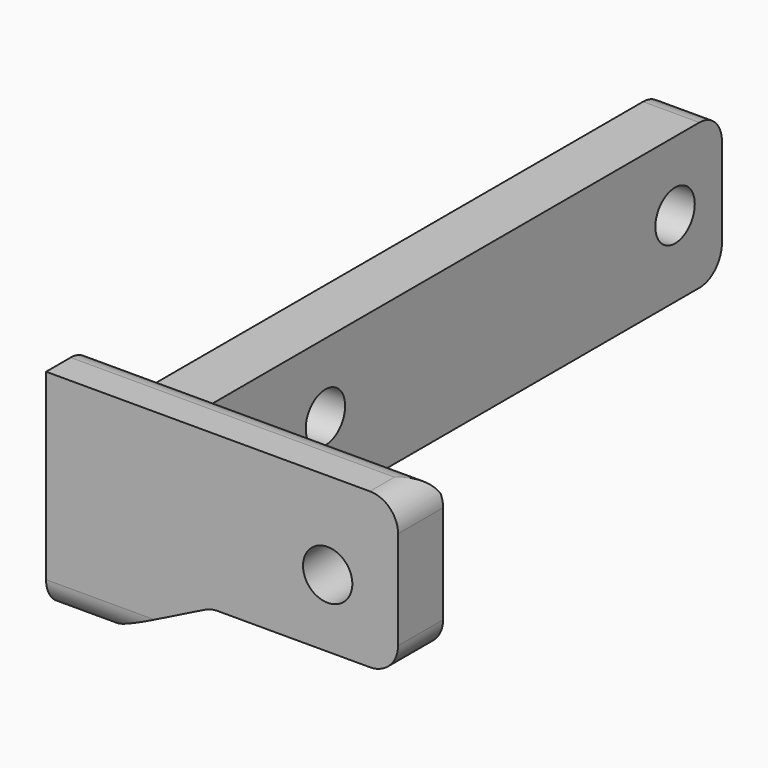
from build123d import *

# Parameters (mm, degrees)
F0_W         = 4
F0_H         = 51
F0_H_2       = 4
F0_W_2       = 21
F1_DEPTH     = 15
F4_D         = 3.5
F4_ON_F3_D   = 3.5
F5_DEPTH     = 25
F6_DEPTH     = 25
F7_T1_DEPTH  = 4
F7_T3_DEPTH  = 14
F7_T5_DEPTH  = 13.3694414049
F7_T7_DEPTH  = 14
F7_T9_DEPTH  = 30.9469097591
F7_T11_DEPTH = 13.6920837807


# Not quite as in the source:
# - a fillet or chamfer that OpenCascade refuses, or shapes differently, is made with other operations: its cross-section is extruded or revolved along the edge and cut away or added


with BuildPart() as f1:
    # F0 (on Top) → F1 (new body)
    with BuildSketch(Plane.XY):
        with Locations((0, 2)):
            Rectangle(F0_W, F0_H)
        with Locations((0, -25.5)):
            Rectangle(F0_W, F0_H_2)
        with Locations((12.5, -25.5)):
            Rectangle(F0_W_2, F0_H_2)
    extrude(amount=F1_DEPTH)

    # F4 (through all)
    with Locations(Plane(origin=(-2, 0, 0), x_dir=(0, -1, 0), z_dir=(-1, 0, 0))):
        with Locations((-23.34, 5.4024579003), (7.7, 5.4024579003)):
            Hole(F4_D / 2)

    # F4 on F3 (through all)
    with Locations(Plane.XZ.offset(27.5)):
        with Locations((18, 8.8024579003)):
            Hole(F4_ON_F3_D / 2)

    # F2 (on face) → F5 (cut)
    with BuildSketch(Plane(origin=(-2, 0, 0), x_dir=(0, -1, 0), z_dir=(-1, 0, 0))):
        Polygon((-27.5, 15), (-27.5, 10.3389231786), (21.5976021229, 10.3389231786), (24.1305585951, 15), align=None)
    extrude(amount=-F5_DEPTH, mode=Mode.SUBTRACT)

    # F3 (on face) → F6 (cut)
    with BuildSketch(Plane.XZ.offset(27.5)):
        Polygon((23, 0), (23, 4), (9.7110802308, 4), (1.6920837807, 0), align=None)
    extrude(amount=-F6_DEPTH, mode=Mode.SUBTRACT)

    # F7: fillet of radius 2 on 7 edges, made by hand

    # F7_s2 → F7_t1 (join)
    with BuildSketch(Plane.XZ.offset(23.5)):
        with BuildLine():
            ThreePointArc((9.2894845277, 3.7897015141), (9.7236323162, 3.9467155709), (10.1822154449, 4))
            Line((10.1822154449, 4), (9.7110802308, 4))
            Line((9.7110802308, 4), (9.2894845277, 3.7897015141))
        make_face()
    extrude(amount=F7_T1_DEPTH)

    # F7_s4 → F7_t3 (cut)
    with BuildSketch(Plane.YZ.offset(-7)):
        with BuildLine():
            ThreePointArc((27.5, 8.3389231786), (26.9142135624, 9.753136741), (25.5, 10.3389231786))
            Line((25.5, 10.3389231786), (27.5, 10.3389231786))
            Line((27.5, 10.3389231786), (27.5, 8.3389231786))
        make_face()
        with BuildLine():
            ThreePointArc((27.5, 2), (26.9142135624, 0.5857864376), (25.5, 0))
            Line((25.5, 0), (27.5, 0))
            Line((27.5, 0), (27.5, 2))
        make_face()
    extrude(amount=F7_T3_DEPTH, mode=Mode.SUBTRACT)

    # F7_s6 → F7_t5 (cut)
    with BuildSketch(Plane.XZ.offset(19.1305585951)):
        with BuildLine():
            ThreePointArc((21, 15), (22.4142135624, 14.4142135624), (23, 13))
            Line((23, 13), (23, 15))
            Line((23, 15), (21, 15))
        make_face()
    extrude(amount=F7_T5_DEPTH, mode=Mode.SUBTRACT)

    # F7_s8 → F7_t7 (cut)
    with BuildSketch(Plane.XZ.offset(18.5)):
        with BuildLine():
            ThreePointArc((21, 4), (22.4142135624, 4.5857864376), (23, 6))
            Line((23, 6), (23, 4))
            Line((23, 4), (21, 4))
        make_face()
    extrude(amount=F7_T7_DEPTH, mode=Mode.SUBTRACT)

    # F7_s10 → F7_t9 (cut)
    with BuildSketch(Plane.YZ.offset(-4.9734548795)):
        with BuildLine():
            ThreePointArc((-25.3199405469, 15), (-24.2976673595, 14.7189989908), (-23.5626539694, 13.9549575303))
            Line((-23.5626539694, 13.9549575303), (-24.1305585951, 15))
            Line((-24.1305585951, 15), (-25.3199405469, 15))
        make_face()
    extrude(amount=F7_T9_DEPTH, mode=Mode.SUBTRACT)

    # F7_s12 → F7_t11 (cut)
    with BuildSketch(Plane.YZ.offset(-7)):
        with BuildLine():
            ThreePointArc((-25.5, 0), (-26.9142135624, 0.5857864376), (-27.5, 2))
            Line((-27.5, 2), (-27.5, 0))
            Line((-27.5, 0), (-25.5, 0))
        make_face()
    extrude(amount=F7_T11_DEPTH, mode=Mode.SUBTRACT)


solid = f1.part
